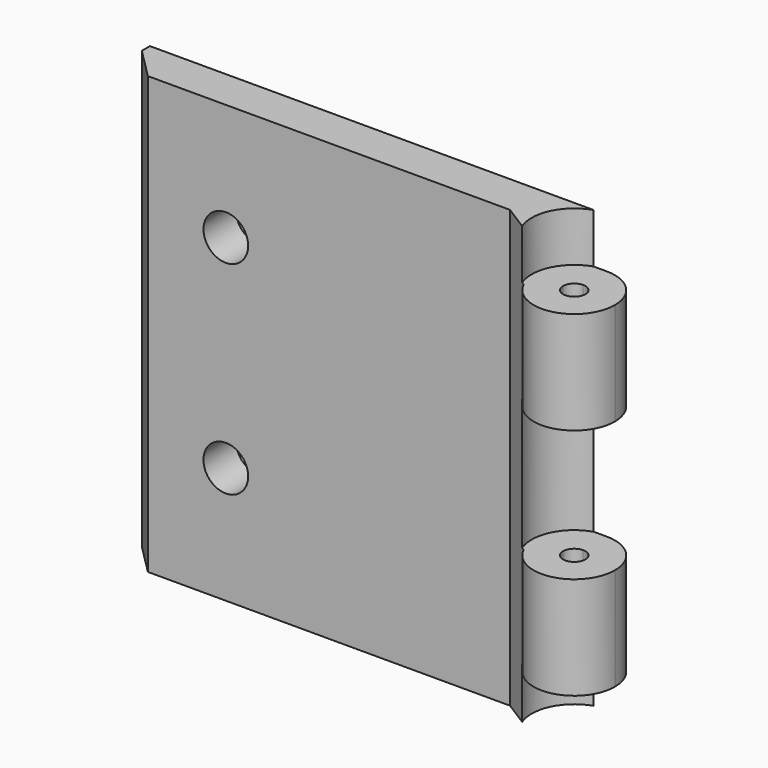
from build123d import *

# Parameters (mm, degrees)
F1_DEPTH    = 43
F2_T1_DEPTH = 43
F2_T3_DEPTH = 58.4300979278
F4_D        = 4.4
F5_R        = 4.2
F6_DEPTH    = 5
F7_START    = 15.1
F7_DEPTH    = 12.9
F8_START    = 38.1
F8_DEPTH    = 11.9


# Not quite as in the source:
# - a fillet or chamfer that OpenCascade refuses, or shapes differently, is made with other operations: its cross-section is extruded or revolved along the edge and cut away or added


with BuildPart() as f1:
    # F0 (on Top) → F1 (new body)
    with BuildSketch(Plane.XY):
        with BuildLine():
            Line((-22.5, -2), (18.5, -2))
            ThreePointArc((18.5, -2), (19.6715728753, 0.8284271247), (22.5, 2))
            Line((22.5, 2), (-22.5, 2))
            Line((-22.5, 2), (-22.5, -2))
        make_face()
        with BuildLine():
            Line((18.5, -2), (21.4, -2))
            ThreePointArc((21.4, -2), (21.7221825407, -1.2221825407), (22.5, -0.9))
            Line((22.5, -0.9), (22.5, 2))
            ThreePointArc((22.5, 2), (19.6715728753, 0.8284271247), (18.5, -2))
        make_face()
        with BuildLine():
            ThreePointArc((23.6, -2), (22.5, -3.1), (21.4, -2))
            Line((21.4, -2), (18.5, -2))
            ThreePointArc((18.5, -2), (22.5, -6), (26.5, -2))
            ThreePointArc((26.5, -2), (25.3284271247, 0.8284271247), (22.5, 2))
            Line((22.5, 2), (22.5, -0.9))
            ThreePointArc((22.5, -0.9), (23.2778174593, -1.2221825407), (23.6, -2))
        make_face()
    extrude(amount=F1_DEPTH)

    # F2: chamfer of 3 on 2 edges, made by hand

    # F2_s2 → F2_t1 (join)
    with BuildSketch(Plane.XY):
        with BuildLine():
            Line((16.0740261691, -1.9358573019), (18.9873868989, -3.7784284123))
            Line((18.9873868989, -3.7784284123), (19.0415973731, -3.7527141266))
            ThreePointArc((19.0415973731, -3.7527141266), (18.6659635809, -2.9076148618), (18.56, -2))
            Line((18.56, -2), (18.5, -1.94))
            ThreePointArc((18.5, -1.94), (17.2870130845, -1.94), (16.0740261691, -1.8758573019))
            Line((16.0740261691, -1.8758573019), (16.0740261691, -1.9358573019))
        make_face()
    extrude(amount=F2_T1_DEPTH)

    # F2_s4 → F2_t3 (cut)
    with BuildSketch(Plane.XY.offset(-7.7150489639)):
        with BuildLine():
            Line((-22.5848528137, 1.0848528137), (-19.4151471863, -2.0848528137))
            Line((-19.4151471863, -2.0848528137), (-19.4151471863, -2.1448528137))
            ThreePointArc((-19.4151471863, -2.1448528137), (-20.9575735931, -2.06), (-22.5, -2.06))
            Line((-22.5, -2.06), (-22.56, -2))
            ThreePointArc((-22.56, -2), (-22.56, -0.4575735931), (-22.6448528137, 1.0848528137))
            Line((-22.6448528137, 1.0848528137), (-22.5848528137, 1.0848528137))
        make_face()
    extrude(amount=F2_T3_DEPTH, mode=Mode.SUBTRACT)

    # F4 (through all)
    with Locations(Plane.XZ.offset(2)):
        with Locations((-11.8245553203, 31.5), (-11.8245553203, 11.5)):
            Hole(F4_D / 2)

    # F5 (on face) → F6 (cut)
    with BuildSketch(Plane.XY):
        with Locations((22.5, -2)):
            Circle(F5_R)
    extrude(amount=F6_DEPTH, mode=Mode.SUBTRACT)

    # F5 (on face) → F7 (cut)
    with BuildSketch(Plane.XY.offset(F7_START)):
        with Locations((22.5, -2)):
            Circle(F5_R)
    extrude(amount=F7_DEPTH, mode=Mode.SUBTRACT)

    # F5 (on face) → F8 (cut)
    with BuildSketch(Plane.XY.offset(F8_START)):
        with Locations((22.5, -2)):
            Circle(F5_R)
    extrude(amount=F8_DEPTH, mode=Mode.SUBTRACT)


solid = f1.part
